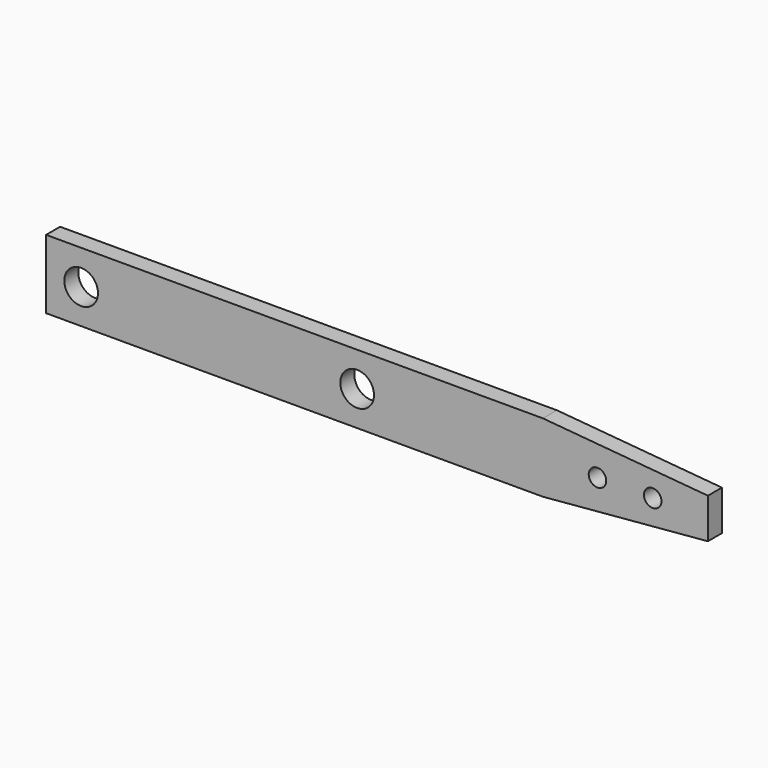
from build123d import *

# Parameters (mm, degrees)
F0_R     = 3.0502649117
F0_R_2   = 1.5875
F1_DEPTH = 3.175


# Not quite as in the source:
# - a length typed as a fraction of an inch, garbled in the dataset ("3 / 203.2 mm" for 3/8 in), is restored


with BuildPart() as f1:
    # F0 (on Front) → F1 (new body)
    with BuildSketch(Plane.XZ):
        Polygon((53.3261225373, -2.7374546753), (-36.6738774627, -2.7374546753), (-36.6738774627, -15.2374546753), (53.3261225373, -15.2374546753), (83.21196348, -12.6227823928), (83.21196348, -8.9778823928), (83.21196348, -5.3521269577), align=None)
        with Locations((-30.3238774627, -8.9874546753)):
            Circle(F0_R, mode=Mode.SUBTRACT)
        with Locations((19.6761225373, -8.9874546753)):
            Circle(F0_R, mode=Mode.SUBTRACT)
        with Locations((63.21196348, -8.9778823928)):
            Circle(F0_R_2, mode=Mode.SUBTRACT)
        with Locations((73.21196348, -8.9778823928)):
            Circle(F0_R_2, mode=Mode.SUBTRACT)
    extrude(amount=F1_DEPTH)


solid = f1.part
